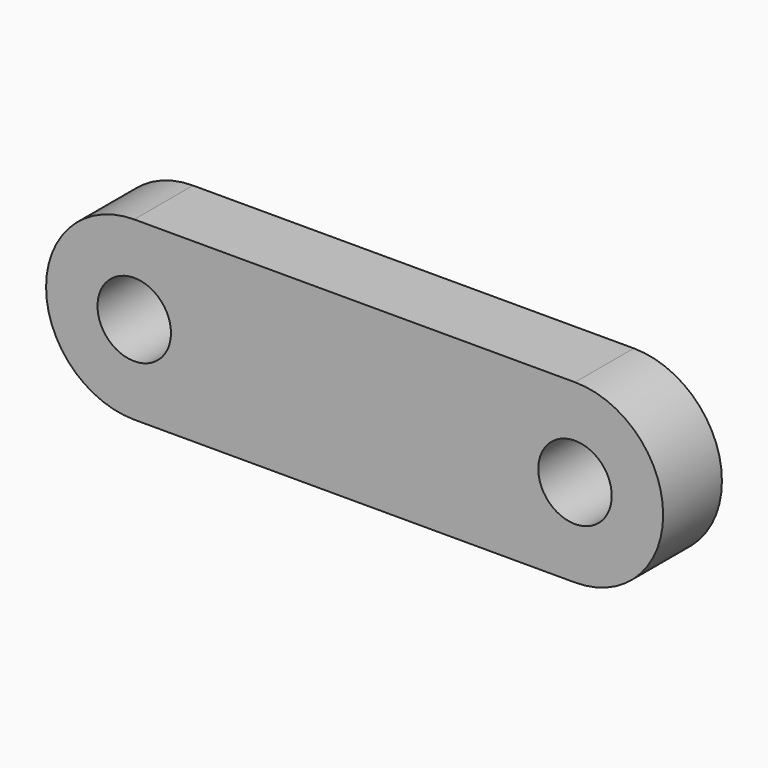
from build123d import *

# Parameters (mm, degrees)
F0_R     = 2.5
F1_DEPTH = 5


# Not quite as in the source:
# - a feature names something its author has since deleted; it is built from what else it names


with BuildPart() as f1:
    # F0 (on Front) → F1 (new body)
    with BuildSketch(Plane.XZ):
        with BuildLine():
            ThreePointArc((0, 12), (-6, 6), (0, 0))
            Line((0, 0), (30, 0))
            ThreePointArc((30, 0), (36, 6), (30, 12))
            Line((30, 12), (0, 12))
        make_face()
        with Locations((0, 6)):
            Circle(F0_R, mode=Mode.SUBTRACT)
        with Locations((30, 6)):
            Circle(F0_R, mode=Mode.SUBTRACT)
    extrude(amount=F1_DEPTH)


solid = f1.part
